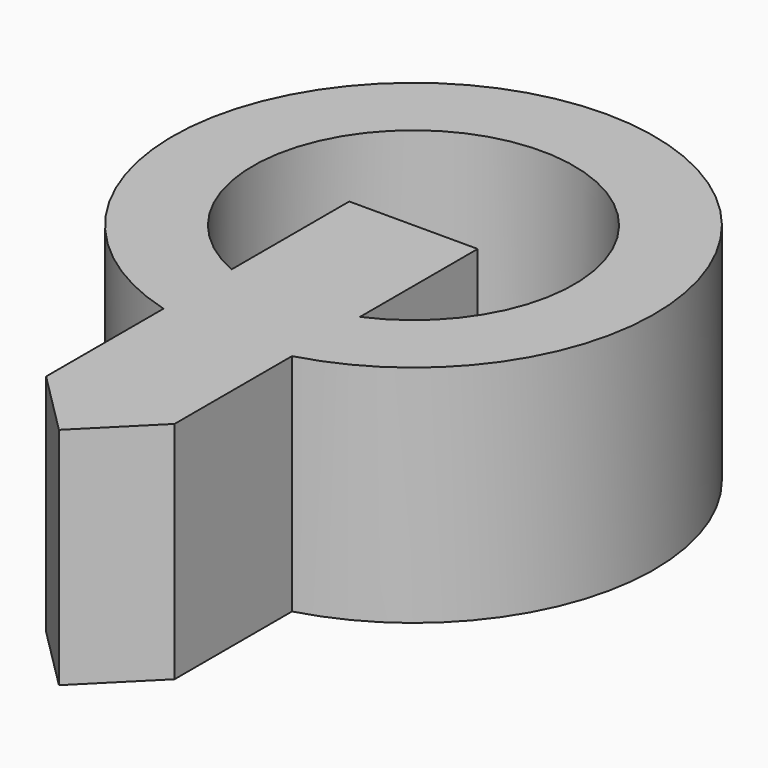
from build123d import *

# Parameters (mm, degrees)
F0_R     = 37.5
F0_R_2   = 25
F1_DEPTH = 35
F2_W     = 20
F2_H     = 35
F3_DEPTH = 69
F4_SIZE  = 9.99999


# Not quite as in the source:
# - a fillet or chamfer is up to 0.001 mm smaller than in the source, because OpenCascade refuses the exact size


with BuildPart() as f1:
    # F0 (on Top) → F1 (new body)
    with BuildSketch(Plane.XY):
        Circle(F0_R)
        Circle(F0_R_2, mode=Mode.SUBTRACT)
    extrude(amount=F1_DEPTH)

    # F2 (on Front) → F3 (join)
    with BuildSketch(Plane.XZ):
        with Locations((0, 17.5)):
            Rectangle(F2_W, F2_H)
    extrude(amount=F3_DEPTH)

    # F4 (size 10 in the source; OpenCascade refuses exactly that, so slightly less here)
    f4_edges = [f1.edges().sort_by_distance(p)[0] for p in [
        (-10, -69, 17.5),
        (10, -69, 17.5),
    ]]
    chamfer(f4_edges, length=F4_SIZE)


solid = f1.part
